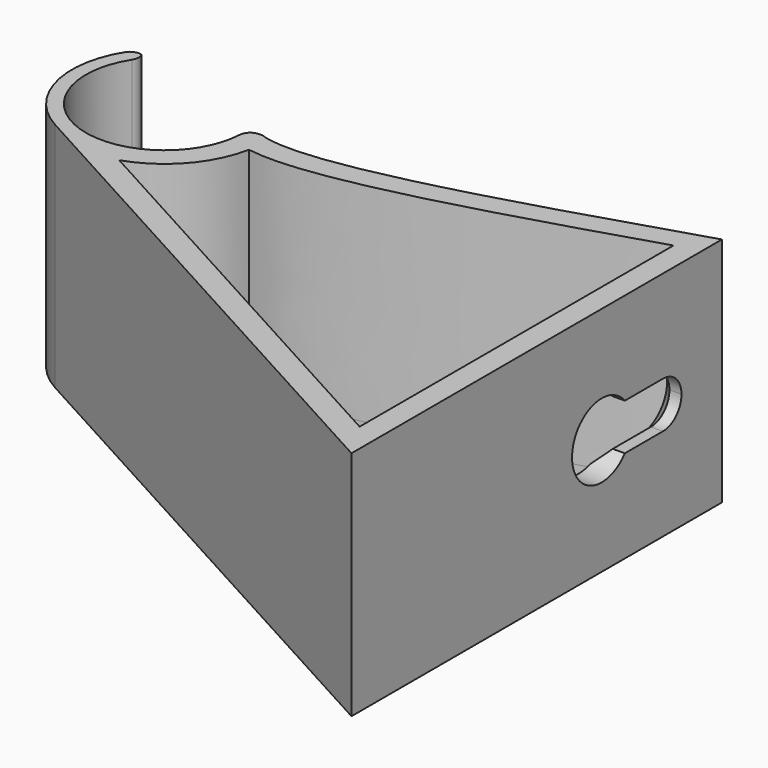
from build123d import *

# Parameters (mm, degrees)
F1_DEPTH    = 25
F2_T1_DEPTH = 30.6274350033
F2_T3_DEPTH = 31.8341602247
F3_T        = -2.5
F4_DEPTH    = 25
F6_DEPTH    = 3
F7_SIZE     = 1.2


# Not quite as in the source:
# - a fillet or chamfer that OpenCascade refuses, or shapes differently, is made with other operations: its cross-section is extruded or revolved along the edge and cut away or added


with BuildPart() as f1:
    # F0 (on Top) → F1 (new body)
    with BuildSketch(Plane.XY):
        with BuildLine():
            Line((0, -23.9775525033), (0, 0))
            Line((0, 0), (0, 26.0224474967))
            add(Edge.make_bspline(
                [(0, 26.0224474967), (-18.2413181838, 20.2646104982), (-36.4872975651, 14.5034889639), (-42.1967271812, 16.6896569806)],
                knots=[0, 0, 0, 0, 0.7457520739, 0.7457520739, 0.7457520739, 0.7457520739], degree=3))
            ThreePointArc((-42.1967271812, 16.6896569806), (-46.7941768856, 7.5931695596), (-56.9807893445, 7.2532375123))
            Line((-56.9807893445, 7.2532375123), (0, -23.9775525033))
        make_face()
        with BuildLine():
            ThreePointArc((-56.9807893445, 7.2532375123), (-46.7941768856, 7.5931695596), (-42.1967271812, 16.6896569806))
            Line((-42.1967271812, 16.6896569806), (-43.6933846934, 16.589575558))
            ThreePointArc((-43.6933846934, 16.589575558), (-54.7874105132, 7.9340356852), (-58.7207947374, 21.4441899376))
            Line((-58.7207947374, 21.4441899376), (-59.8760331153, 22.4009680155))
            ThreePointArc((-59.8760331153, 22.4009680155), (-61.9966403153, 14.1450934668), (-56.9807893445, 7.2532375123))
        make_face()
    extrude(amount=F1_DEPTH)

    # F2: fillet of radius 1.2 on 3 edges, made by hand

    # F2_s2 → F2_t1 (cut)
    with BuildSketch(Plane.XY.offset(-2.8137175017)):
        with BuildLine():
            ThreePointArc((-59.3412383143, 20.5926836221), (-59.1675384199, 21.4239873058), (-59.5875985888, 22.1620841304))
            Line((-59.5875985888, 22.1620841304), (-58.7207947374, 21.4441899376))
            ThreePointArc((-58.7207947374, 21.4441899376), (-59.0442222025, 21.0280589954), (-59.3412383143, 20.5926836221))
        make_face()
        with BuildLine():
            ThreePointArc((-42.5704056438, 16.6646691181), (-43.3428946364, 16.3118260592), (-43.6883739189, 15.5360158161))
            ThreePointArc((-43.6883739189, 15.5360158161), (-43.6745400624, 16.0628733972), (-43.6933846934, 16.589575558))
            Line((-43.6933846934, 16.589575558), (-42.5704056438, 16.6646691181))
        make_face()
    extrude(amount=F2_T1_DEPTH, mode=Mode.SUBTRACT)

    # F2_s4 → F2_t3 (cut)
    with BuildSketch(Plane.XY.offset(-3.4170801123)):
        with BuildLine():
            ThreePointArc((-58.8885337226, 21.5831127668), (-59.8476100394, 21.8431932263), (-60.6738896743, 21.2911685965))
            ThreePointArc((-60.6738896743, 21.2911685965), (-60.2939449544, 21.8597159591), (-59.8760331153, 22.4009680155))
            Line((-59.8760331153, 22.4009680155), (-58.8885337226, 21.5831127668))
        make_face()
    extrude(amount=F2_T3_DEPTH, mode=Mode.SUBTRACT)

    # F3
    f3_openings = [f1.faces().sort_by_distance(p)[0] for p in [
        (-19.977186, 3.669983, 25),
    ]]
    offset(amount=F3_T, openings=f3_openings)

    # F4 (cut): a face of the model
    f4_faces = [f1.faces().sort_by_distance(p)[0] for p in [
        (-18.9574034875, 3.5679781743, 2.5),
    ]]
    extrude(f4_faces, amount=-F4_DEPTH, mode=Mode.SUBTRACT)

    # F5 (on face) → F6 (cut)
    with BuildSketch(Plane.YZ):
        with BuildLine():
            ThreePointArc((12.9166145043, 10), (13.5683701333, 11.1752351146), (13.7941155051, 12.5))
            ThreePointArc((13.7941155051, 12.5), (13.5683701333, 13.8247648854), (12.9166145043, 15))
            ThreePointArc((12.9166145043, 15), (5.7941155051, 12.5), (12.9166145043, 10))
        make_face()
        with BuildLine():
            ThreePointArc((20.5641841143, 12.5), (19.8319510673, 14.267766953), (18.0641841143, 15))
            ThreePointArc((18.0641841143, 15), (15.5641841143, 12.5), (18.0641841143, 10))
            ThreePointArc((18.0641841143, 10), (19.8319510673, 10.732233047), (20.5641841143, 12.5))
        make_face()
        with BuildLine():
            ThreePointArc((12.9166145043, 15), (13.5683701333, 13.8247648854), (13.7941155051, 12.5))
            ThreePointArc((13.7941155051, 12.5), (13.5683701333, 11.1752351146), (12.9166145043, 10))
            Line((12.9166145043, 10), (18.0641841143, 10))
            ThreePointArc((18.0641841143, 10), (15.5641841143, 12.5), (18.0641841143, 15))
            Line((18.0641841143, 15), (12.9166145043, 15))
        make_face()
    extrude(amount=-F6_DEPTH, mode=Mode.SUBTRACT)

    # F7
    f7_edges = [f1.edges().sort_by_distance(p)[0] for p in [
        (-2.5, 15.490399, 10),
        (-2.5, 15.490399, 15),
        (-2.5, 20.564184, 12.5),
    ]]
    chamfer(f7_edges, length=F7_SIZE)


solid = f1.part
